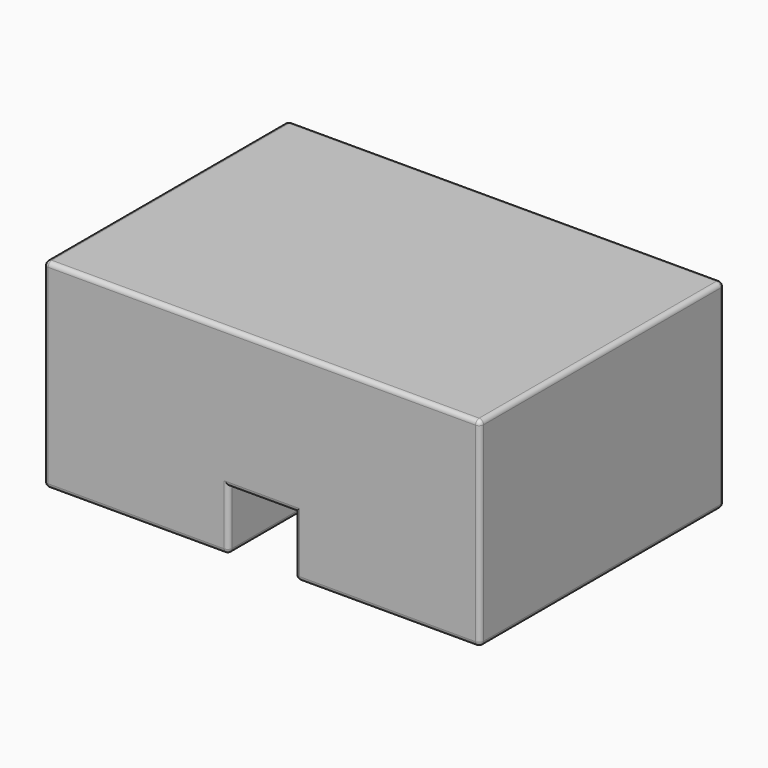
from build123d import *

# Parameters (mm, degrees)
F0_W     = 500.126
F0_H     = 228.6
F1_DEPTH = 350.012
F2_R     = 5.08
F4_DEPTH = 350.013
F5_R     = 5.08


with BuildPart() as f1:
    # F0 (on Front) → F1 (new body)
    with BuildSketch(Plane.XZ):
        Rectangle(F0_W, F0_H)
    extrude(amount=-F1_DEPTH)

    # F2
    f2_edges = [f1.edges().sort_by_distance(p)[0] for p in [
        (0, 0, -114.3),
        (250.063, 0, 0),
        (0, 0, 114.3),
        (-250.063, 0, 0),
        (-250.063, 175.006, 114.3),
        (-250.063, 175.006, -114.3),
        (-250.063, 350.012, 0),
        (250.063, 175.006, 114.3),
        (0, 350.012, 114.3),
        (250.063, 175.006, -114.3),
        (0, 350.012, -114.3),
        (250.063, 350.012, 0),
    ]]
    fillet(f2_edges, radius=F2_R)

    # F3 (on face) → F4 (cut, through all)
    with BuildSketch(Plane(origin=(0, 350.012, 0), x_dir=(-1, 0, 0), z_dir=(0, 1, 0))):
        Polygon((38.1, -94.107), (38.1, -45.6269201875), (0, -45.6269201875), (-38.1, -45.6269201875), (-38.1, -121.8269201875), (0, -121.8269201875), (38.1, -121.8269201875), align=None)
    extrude(amount=-F4_DEPTH, mode=Mode.SUBTRACT)

    # F5
    f5_edges = [f1.edges().sort_by_distance(p)[0] for p in [
        (0, 0, -45.62692),
        (-38.1, 0, -77.42346),
        (38.1, 0, -77.42346),
        (-38.1, 350.012, -77.42346),
        (0, 350.012, -45.62692),
        (38.1, 350.012, -77.42346),
        (-38.1, 175.006, -114.3),
        (-38.1, 1.487898, -112.812102),
        (-38.1, 348.524102, -112.812102),
        (38.1, 1.487898, -112.812102),
        (38.1, 348.524102, -112.812102),
        (38.1, 175.006, -114.3),
    ]]
    fillet(f5_edges, radius=F5_R)


solid = f1.part
